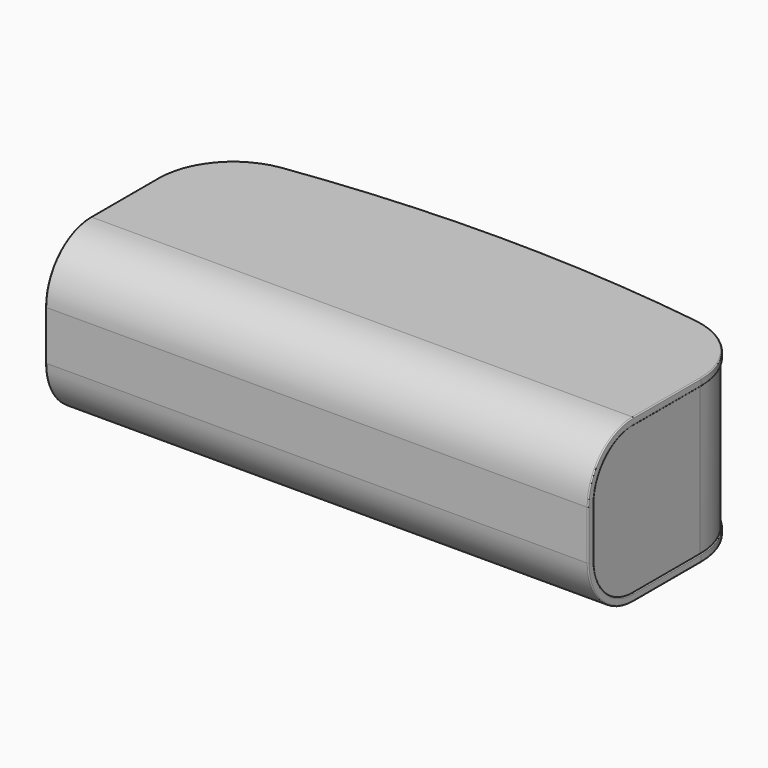
from build123d import *

# Parameters (mm, degrees)
F0_W     = 220
F0_H     = 80
F1_DEPTH = 60
F2_R     = 30
F3_R     = 20
F5_DEPTH = 0.4
F6_DEPTH = 220.4
F9_DEPTH = 66
F10_R    = 0.4


with BuildPart() as f1:
    # F0 (on Top) → F1 (new body)
    with BuildSketch(Plane.XY):
        Rectangle(F0_W, F0_H)
        with BuildLine():
            Line((-110, 40), (110, 40))
            ThreePointArc((110, 40), (0, 50), (-110, 40))
        make_face()
    extrude(amount=F1_DEPTH)

    # F2
    f2_edges = [f1.edges().sort_by_distance(p)[0] for p in [
        (-110, 40, 30),
        (110, 40, 30),
    ]]
    fillet(f2_edges, radius=F2_R)

    # F3
    f3_edges = [f1.edges().sort_by_distance(p)[0] for p in [
        (0, -40, 60),
        (0, -40, 0),
    ]]
    fillet(f3_edges, radius=F3_R)


with BuildPart() as f5:
    # F4 (on face) → F5 (new body)
    with BuildSketch(Plane.YZ.offset(110)):
        with BuildLine():
            Line((-20, -3), (14.4562646538, -3))
            Line((14.4562646538, -3), (50.4, -3))
            Line((50.4, -3), (50.4, 0))
            Line((50.4, 0), (50, 0))
            Line((50, 0), (44.1695197221, 0))
            Line((44.1695197221, 0), (14.4562646538, 0))
            Line((14.4562646538, 0), (-20, 0))
            ThreePointArc((-20, 0), (-34.1421356237, 5.8578643763), (-40, 20))
            Line((-40, 20), (-40, 40))
            ThreePointArc((-40, 40), (-34.1421356237, 54.1421356237), (-20, 60))
            Line((-20, 60), (14.4562646538, 60))
            Line((14.4562646538, 60), (44.1695197221, 60))
            Line((44.1695197221, 60), (50, 60))
            Line((50, 60), (50.4, 60))
            Line((50.4, 60), (50.4, 63))
            Line((50.4, 63), (14.4562646538, 63))
            Line((14.4562646538, 63), (-20, 63))
            ThreePointArc((-20, 63), (-36.2634559673, 56.2634559673), (-43, 40))
            Line((-43, 40), (-43, 20))
            ThreePointArc((-43, 20), (-36.2634559673, 3.7365440327), (-20, -3))
        make_face()
    extrude(amount=F5_DEPTH)

    # F6 (add): a face of the model
    f6_faces = [f5.faces().sort_by_distance(p)[0] for p in [
        (110, -35.4547669047, 55.4547669047),
    ]]
    extrude(f6_faces, amount=F6_DEPTH)

    # F7: union 

    # F8 (on face) → F9 (cut, through all)
    with BuildSketch(Plane.XY.offset(63)):
        with BuildLine():
            Line((-110.4, 50.4), (-110.4, 14.4562646538))
            ThreePointArc((-110.4, 14.4562646538), (-102.9306600955, 34.4148424485), (-84.1931034483, 44.5656964563))
            ThreePointArc((-84.1931034483, 44.5656964563), (-42.1975051576, 48.9396772739), (0, 50.4))
            Line((0, 50.4), (-110.4, 50.4))
        make_face()
        with BuildLine():
            Line((110.4, 50.4), (0, 50.4))
            ThreePointArc((0, 50.4), (42.1975051575, 48.9396772739), (84.1931034483, 44.5656964563))
            ThreePointArc((84.1931034483, 44.5656964563), (102.9306600955, 34.4148424485), (110.4, 14.4562646538))
            Line((110.4, 14.4562646538), (110.4, 50.4))
        make_face()
    extrude(amount=-F9_DEPTH, mode=Mode.SUBTRACT)

    # F10
    f10_edges = [f5.edges().sort_by_distance(p)[0] for p in [
        (110.4, -2.771868, 63),
        (110.4, 14.456265, 61.5),
        (110.4, -2.771868, 60),
        (110.4, -34.142136, 54.142136),
        (110.4, -40, 30),
        (110.4, -34.142136, 5.857864),
        (110.4, -2.771868, 0),
        (110.4, 14.456265, -1.5),
        (110.4, -2.771868, -3),
        (110.4, -36.263456, 3.736544),
        (110.4, -43, 30),
        (110.4, -36.263456, 56.263456),
        (102.93066, 34.414842, 0),
        (102.93066, 34.414842, -3),
        (84.193103, 44.565696, -1.5),
        (102.93066, 34.414842, 63),
        (102.93066, 34.414842, 60),
        (84.193103, 44.565696, 61.5),
        (-102.93066, 34.414842, 0),
        (-84.193103, 44.565696, -1.5),
        (-102.93066, 34.414842, -3),
        (-110.4, 14.456265, -1.5),
        (-102.93066, 34.414842, 63),
        (-84.193103, 44.565696, 61.5),
        (-102.93066, 34.414842, 60),
        (-110.4, 14.456265, 61.5),
        (-110.4, -2.771868, 63),
        (-110.4, -2.771868, 60),
        (-110.4, -34.142136, 54.142136),
        (-110.4, -40, 30),
        (-110.4, -34.142136, 5.857864),
        (-110.4, -2.771868, 0),
        (-110.4, -2.771868, -3),
        (-110.4, -36.263456, 3.736544),
        (-110.4, -43, 30),
        (-110.4, -36.263456, 56.263456),
        (0, 50.4, -3),
        (0, 50.4, 0),
        (0, 50.4, 60),
        (0, 50.4, 63),
    ]]
    fillet(f10_edges, radius=F10_R)


solid = Compound([f1.part, f5.part])
